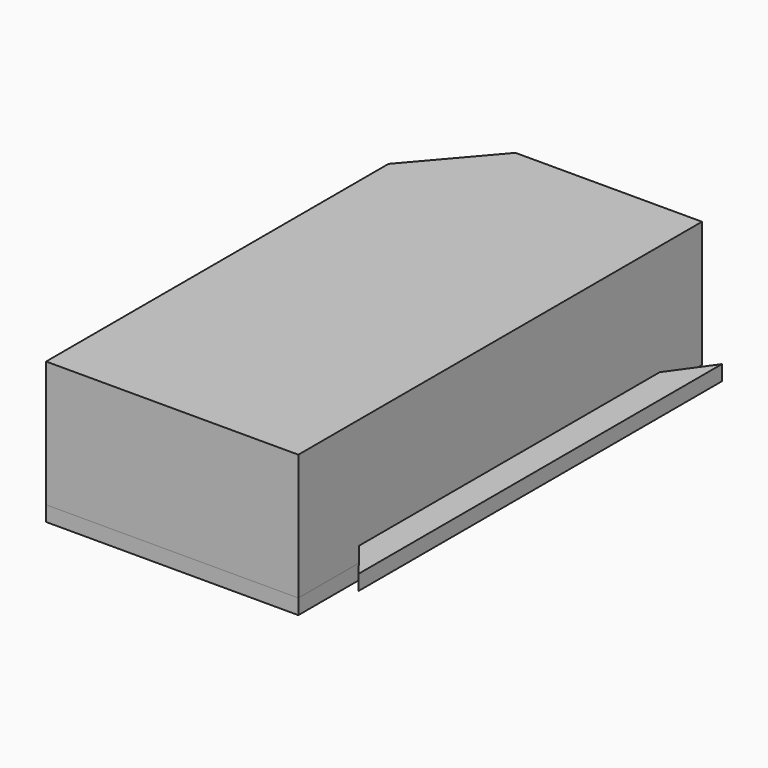
from build123d import *

# Parameters (mm, degrees)
F0_W      = 50
F0_H      = 100
F1_DEPTH  = 3
F3_DEPTH  = 3
F6_DEPTH  = 3
F8_DEPTH  = 25
F12_DEPTH = 25


# Not quite as in the source:
# - a feature of the source that left no trace in its solid (it failed there, or was rolled back) is left out


with BuildPart() as f1:
    # F0 (on Top) → F1 (new body)
    with BuildSketch(Plane.XY):
        with Locations((0.0869164988, -0.3243560148)):
            Rectangle(F0_W, F0_H)
    extrude(amount=F1_DEPTH)

    # F4 (on face) → F6 (cut)
    with BuildSketch(Plane.XY.offset(3)):
        Polygon((-24.9130835012, 49.6756439852), (-24.9130835012, 34.5086446194), (-11.8761310107, 49.6756439852), align=None)
    extrude(amount=-F6_DEPTH, mode=Mode.SUBTRACT)

    # F7 (on face) → F8 (cut)
    with BuildSketch(Plane.XY.offset(3)):
        Polygon((25.0869164988, 49.6756439852), (11.2441298249, 49.6756439852), (25.0869164988, 32.1048707049), align=None)
    extrude(amount=-F8_DEPTH, mode=Mode.SUBTRACT)


with BuildPart() as f3:
    # F2 (on face) → F3 (new body)
    with BuildSketch(Plane.XY.offset(3)):
        Polygon((30.9052136403, 47.3424089814), (25.0869164988, 39.2093026638), (25.0869164988, -35.3014330966), (30.9052136403, -42.6575910186), align=None)
    extrude(amount=F3_DEPTH)


with BuildPart() as f12:
    # F10 (on face) → F12 (new body)
    with BuildSketch(Plane.XY.offset(3)):
        with BuildLine():
            add(Edge.make_bspline(
                [(0, 30), (-5.1961524227, 30), (-2.5980762114, -15), (0, -60), (2.5980762114, -15), (5.1961524227, 30), (0, 30)],
                knots=[0, 0, 0, 2.0943951024, 2.0943951024, 4.1887902048, 4.1887902048, 6.2831853072, 6.2831853072, 6.2831853072], degree=2, weights=[1, 0.5, 1, 0.5, 1, 0.5, 1]))
        make_face()
    extrude(amount=F12_DEPTH)


with BuildPart() as f12b:
    # F9 (on face) → F12, piece 2 (new body)
    with BuildSketch(Plane.XY.offset(3)):
        Polygon((25.0869164988, -50.3243560148), (25.0869164988, 49.6756439852), (-11.8761310107, 49.6756439852), (-24.9130835012, 34.5086446194), (-24.9130835012, -50.3243560148), align=None)
    extrude(amount=F12_DEPTH)


solid = Compound([f1.part, f3.part, f12.part, f12b.part])
